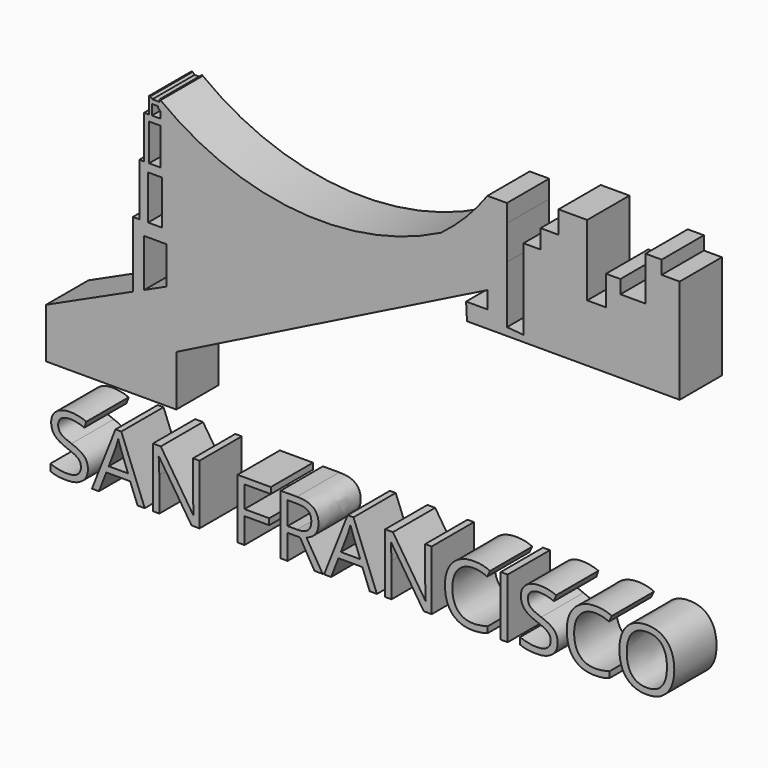
from build123d import *

# Parameters (mm, degrees)
F0_W         = 9.2410445213
F0_H         = 8.2788538177
F0_H_2       = 7.8929657128
F0_W_2       = 0.2195239067
F0_H_3       = 0.2979133278
F0_TEXT_SIZE = 39.5330162456
F1_DEPTH     = 25


# Not quite as in the source:
# - Text() gives the source's letters only with a copy of the font that has no kerning and outlines rounded to 1/6400 em; it was checked with that copy


with BuildPart() as f1:
    # F0 (on Front) → F1 (new body)
    with BuildSketch(Plane.XZ):
        Polygon((-300, -118.6617910862), (-300, -142.2894176923), (-286.4133888585, -142.2894176923), (-254.5032654164, -126.3304831355), (-250.9303432137, -124.5435883993), (-242.9333647605, -120.5441286035), (-242.9333647605, -92.5320801376), (-253.5278499126, -97.3830904261), (-258.8936553192, -99.8399891672), align=None)
        Polygon((-254.5032654164, -126.3304831355), (-286.4133888585, -142.2894176923), (-254.5032654164, -142.2894176923), align=None)
        Polygon((-254.5032654164, -126.3304831355), (-254.5032654164, -142.2894176923), (-250.9303432137, -142.2894176923), (-250.9303432137, -124.5435883993), align=None)
        Polygon((-258.8936553192, -68.685144186), (-258.8936553192, -99.8399891672), (-253.5278499126, -97.3830904261), (-253.5278499126, -74.8785436153), (-242.9333647605, -74.8785436153), (-242.9333647605, -92.5320801376), (-238.3394867645, -90.4286320604), (-238.3394867645, -68.685144186), (-239.9274855852, -68.685144186), (-242.9333647605, -68.685144186), (-245.146766305, -68.685144186), (-251.7026364803, -68.685144186), (-255.8745443821, -68.685144186), align=None)
        Polygon((-250.9303432137, -124.5435883993), (-250.9303432137, -142.2894176923), (-242.9333647605, -142.2894176923), (-242.9333647605, -120.5441286035), align=None)
        Polygon((-242.9333647605, -120.5441286035), (-242.9333647605, -142.2894176923), (-238.3394867645, -142.2894176923), (-238.3394867645, -118.2466320604), align=None)
        Polygon((-242.9333647605, -92.5320801376), (-242.9333647605, -120.5441286035), (-238.3394867645, -118.2466320604), (-238.3394867645, -90.4286320604), align=None)
        Polygon((-255.8745443821, -43.849285692), (-255.8745443821, -68.685144186), (-251.7026364803, -68.685144186), (-251.7026364803, -47.782804817), (-245.146766305, -47.782804817), (-245.146766305, -68.685144186), (-242.9333647605, -68.685144186), (-239.9274855852, -68.685144186), (-239.9274855852, -43.849285692), (-242.9333647605, -43.849285692), (-245.146766305, -43.849285692), (-245.8086758852, -43.849285692), (-251.2171268463, -43.849285692), (-253.5278499126, -43.849285692), align=None)
        Polygon((-238.3394867645, -90.4286320604), (-238.3394867645, -118.2466320604), (-149.8635115183, -73.9979063741), (-91.0160690546, -44.5670430051), (-91.0160690546, -29.9289487302), (-91.0160690546, -21.6500949126), (-94.4814607501, -23.3832113445), (-169.006600976, -58.6824417114), (-237.2701615095, -89.939008663), align=None)
        with BuildLine():
            Line((-238.3394867645, -68.685144186), (-238.3394867645, -90.4286320604))
            Line((-238.3394867645, -90.4286320604), (-237.2701615095, -89.939008663))
            Line((-237.2701615095, -89.939008663), (-169.006600976, -58.6824417114))
            Line((-169.006600976, -58.6824417114), (-94.4814607501, -23.3832113445))
            Line((-94.4814607501, -23.3832113445), (-91.0160690546, -21.6500949126))
            Line((-91.0160690546, -21.6500949126), (-91.0160690546, -13.7571291998))
            Line((-91.0160690546, -13.7571291998), (-91.0160690546, -13.5575999663))
            ThreePointArc((-91.0160690546, -13.5575999663), (-101.6203208989, -21.2604295813), (-112.97141205, -27.8130222692))
            ThreePointArc((-112.97141205, -27.8130222692), (-180.7255321015, -48.4113005262), (-245.8086758852, -20.4990407408))
            Line((-245.8086758852, -20.4990407408), (-245.8086758852, -23.4950948507))
            Line((-245.8086758852, -23.4950948507), (-242.9333647605, -23.4950948507))
            Line((-242.9333647605, -23.4950948507), (-242.9333647605, -43.849285692))
            Line((-242.9333647605, -43.849285692), (-239.9274855852, -43.849285692))
            Line((-239.9274855852, -43.849285692), (-239.9274855852, -68.685144186))
            Line((-239.9274855852, -68.685144186), (-238.3394867645, -68.685144186))
        make_face()
        Polygon((-253.5278499126, -23.4950948507), (-253.5278499126, -43.849285692), (-251.2171268463, -43.849285692), (-251.2171268463, -26.4117624611), (-245.8086758852, -26.4117624611), (-245.8086758852, -43.849285692), (-245.146766305, -43.849285692), (-242.9333647605, -43.849285692), (-242.9333647605, -23.4950948507), (-245.8086758852, -23.4950948507), (-247.01577425, -23.4950948507), (-249.8767524958, -23.4950948507), (-251.2171268463, -23.4950948507), align=None)
        Polygon((-81.7750245333, -44.5670430051), (-91.0160690546, -44.5670430051), (-91.0160690546, -52.6497280442), (-91.0160690546, -60.7324130833), (-81.7750245333, -60.7324130833), (-81.7750245333, -57.0344291627), align=None)
        Polygon((-91.0160690546, -29.9289487302), (-91.0160690546, -44.5670430051), (-81.7750245333, -40.1899729532), (-81.7750245333, -29.9289487302), align=None)
        Polygon((-81.7750245333, -40.1899729532), (-91.0160690546, -44.5670430051), (-81.7750245333, -44.5670430051), align=None)
        Polygon((-91.0160690546, -60.7324130833), (-91.0160690546, -52.6497280442), (-101.13389045, -52.6497280442), (-100.7095724344, -60.7324130833), align=None)
        with Locations((-86.3955467939, -25.7895218214)):
            Rectangle(F0_W, F0_H)
        with BuildLine():
            Line((-251.2171268463, -16.6481509805), (-251.2171268463, -23.4950948507))
            Line((-251.2171268463, -23.4950948507), (-249.8767524958, -23.4950948507))
            Line((-249.8767524958, -23.4950948507), (-249.8767524958, -18.6579637229))
            Line((-249.8767524958, -18.6579637229), (-247.7144939861, -18.6579637229))
            ThreePointArc((-247.7144939861, -18.6579637229), (-248.707928124, -17.6597876258), (-249.6876516591, -16.6481509805))
            Line((-249.6876516591, -16.6481509805), (-250.5805790424, -16.6481509805))
            Line((-250.5805790424, -16.6481509805), (-251.2171268463, -16.6481509805))
        make_face()
        with Locations((-86.3955467939, -17.7036120562)):
            Rectangle(F0_W, F0_H_2)
        Polygon((-73.9489719272, -57.7123955725), (-81.7750245333, -57.0344291627), (-81.7750245333, -60.7324130833), (-73.9489719272, -60.7324130833), align=None)
        Polygon((-251.2171268463, -15.7015882432), (-251.2171268463, -16.6481509805), (-250.5805790424, -16.6481509805), (-250.5805790424, -15.7801955938), (-250.5805790424, -15.7015882432), (-250.7818639278, -15.7015882432), (-251.0185539722, -15.7015882432), align=None)
        with BuildLine():
            Line((-91.0160690546, -13.5575999663), (-91.0160690546, -13.7571291998))
            Line((-91.0160690546, -13.7571291998), (-81.7750245333, -13.7571291998))
            Line((-81.7750245333, -13.7571291998), (-81.7750245333, -5.2861729637))
            ThreePointArc((-81.7750245333, -5.2861729637), (-86.293112647, -9.5363284484), (-91.0160690546, -13.5575999663))
        make_face()
        Polygon((-73.9489719272, -19.514111802), (-73.9489719272, -57.7123955725), (-73.9489719272, -60.7324130833), (0, -60.7324130833), (0, -11.4434491843), (-8.5341287777, -11.4434491843), (-8.5341287777, -5.0718770362), (-16.180023551, -5.0718770362), (-16.180023551, -25.8856844157), (-28.0736219138, -25.8856844157), (-28.0736219138, -19.514111802), (-34.8699837923, -19.514111802), (-34.8699837923, -33.5315726697), (-43.7901765108, -33.5315726697), (-43.7901765108, 0), (-57.3828630149, 0), (-57.3828630149, -10.5939069763), (-65.8783093095, -10.5939069763), (-65.8783093095, -19.514111802), align=None)
        with BuildLine():
            Line((-250.5805790424, -15.7801955938), (-250.5805790424, -16.6481509805))
            Line((-250.5805790424, -16.6481509805), (-249.6876516591, -16.6481509805))
            ThreePointArc((-249.6876516591, -16.6481509805), (-250.1356069803, -16.1762767208), (-250.5805790424, -15.7015882432))
            Line((-250.5805790424, -15.7015882432), (-250.5805790424, -15.7801955938))
        make_face()
        with BuildLine():
            ThreePointArc((-112.97141205, -27.8130222692), (-101.6203208989, -21.2604295813), (-91.0160690546, -13.5575999663))
            Line((-91.0160690546, -13.5575999663), (-91.0160690546, -5.2861729637))
            ThreePointArc((-91.0160690546, -5.2861729637), (-101.1305815694, -17.3908582505), (-112.97141205, -27.8130222692))
        make_face()
        with BuildLine():
            Line((-91.0160690546, -5.2861729637), (-91.0160690546, -13.5575999663))
            ThreePointArc((-91.0160690546, -13.5575999663), (-86.293112647, -9.5363284484), (-81.7750245333, -5.2861729637))
            Line((-81.7750245333, -5.2861729637), (-91.0160690546, -5.2861729637))
        make_face()
        with BuildLine():
            Line((-247.01577425, -18.6579637229), (-247.01577425, -19.3439659228))
            ThreePointArc((-247.01577425, -19.3439659228), (-246.4145620721, -19.9239455928), (-245.8086758852, -20.4990407408))
            Line((-245.8086758852, -20.4990407408), (-245.8086758852, -16.6481509805))
            Line((-245.8086758852, -16.6481509805), (-246.3624924421, -16.6481509805))
            Line((-246.3624924421, -16.6481509805), (-249.6876516591, -16.6481509805))
            ThreePointArc((-249.6876516591, -16.6481509805), (-248.707928124, -17.6597876258), (-247.7144939861, -18.6579637229))
            Line((-247.7144939861, -18.6579637229), (-247.01577425, -18.6579637229))
        make_face()
        with BuildLine():
            ThreePointArc((-245.8086758852, -20.4990407408), (-180.7255321015, -48.4113005262), (-112.97141205, -27.8130222692))
            ThreePointArc((-112.97141205, -27.8130222692), (-181.1233597062, -40.9529453861), (-245.8086758852, -15.7903656363))
            Line((-245.8086758852, -15.7903656363), (-245.8086758852, -16.6481509805))
            Line((-245.8086758852, -16.6481509805), (-245.8086758852, -20.4990407408))
        make_face()
        Polygon((-246.3624924421, -15.7903656363), (-246.3624924421, -16.6481509805), (-245.8086758852, -16.6481509805), (-245.8086758852, -15.7903656363), (-245.954811573, -15.7903656363), (-246.1743354797, -15.7903656363), align=None)
        with Locations((-246.0645735264, -15.6414089724)):
            Rectangle(F0_W_2, F0_H_3)
        with Locations((-300, -188.2737816391)):
            Text('SAN FRANCISCO', F0_TEXT_SIZE, font='Open Sans', text_align=(TextAlign.LEFT, TextAlign.BOTTOM))
    extrude(amount=F1_DEPTH)


solid = f1.part
